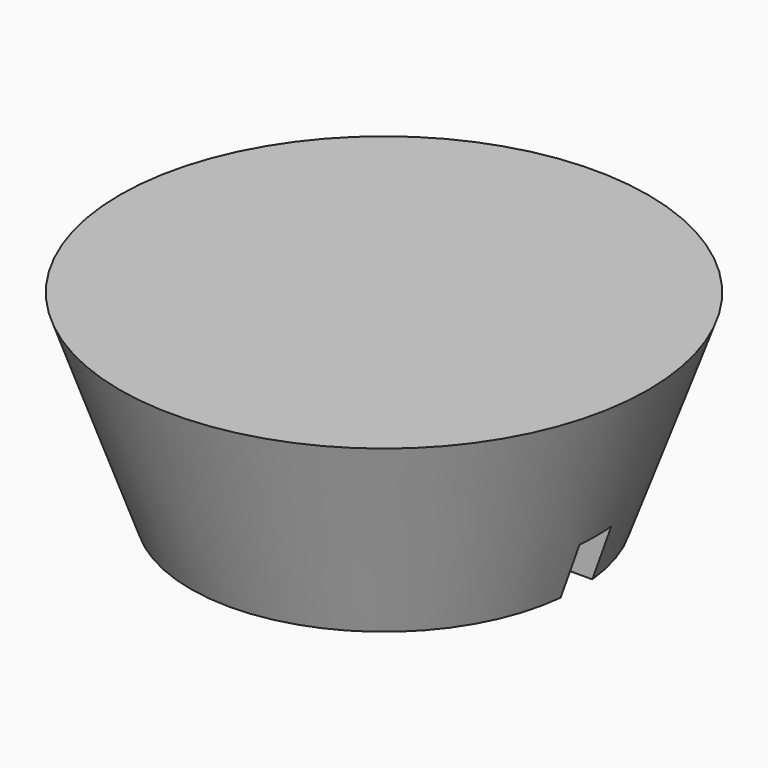
from build123d import *

# Parameters (mm, degrees)
F0_R     = 25.4
F3_R     = 18.6067290317
F8_DEPTH = 5.08
F9_DEPTH = 5.08


# Not quite as in the source:
# - a feature of the source that left no trace in its solid (it failed there, or was rolled back) is left out


with BuildPart() as f4:
    # F0 (on Top) → F4 section 0
    with BuildSketch(Plane.XY):
        Circle(F0_R)
    # F3 (on plane+point) → F4 section 1
    with BuildSketch(Plane.XY.offset(-19.05)):
        Circle(F3_R)
    loft()

    # F5 (on face) → F8 (cut)
    with BuildSketch(Plane(origin=(0, 0, -19.05), x_dir=(1, 0, 0), z_dir=(0, 0, -1))):
        with BuildLine():
            Line((18.5089529757, 1.905), (2.0125971848, 1.905))
            Line((2.0125971848, 1.905), (2.0125971848, 0))
            Line((2.0125971848, 0), (2.0125971848, -1.905))
            Line((2.0125971848, -1.905), (18.5089529757, -1.905))
            ThreePointArc((18.5089529757, -1.905), (18.5822689403, -0.9537537886), (18.6067290317, 0))
            ThreePointArc((18.6067290317, 0), (18.5822689403, 0.9537537886), (18.5089529757, 1.905))
        make_face()
    extrude(amount=-F8_DEPTH, mode=Mode.SUBTRACT)

    # F5 (on face) → F9 (cut)
    with BuildSketch(Plane(origin=(0, 0, -19.05), x_dir=(1, 0, 0), z_dir=(0, 0, -1))):
        with BuildLine():
            Line((26.4462942035, 1.905), (18.5089529757, 1.905))
            ThreePointArc((18.5089529757, 1.905), (18.5822689403, 0.9537537886), (18.6067290317, 0))
            ThreePointArc((18.6067290317, 0), (18.5822689403, -0.9537537886), (18.5089529757, -1.905))
            Line((18.5089529757, -1.905), (26.4462942035, -1.905))
            Line((26.4462942035, -1.905), (26.4462942035, 1.905))
        make_face()
    extrude(amount=-F9_DEPTH, mode=Mode.SUBTRACT)


solid = f4.part
